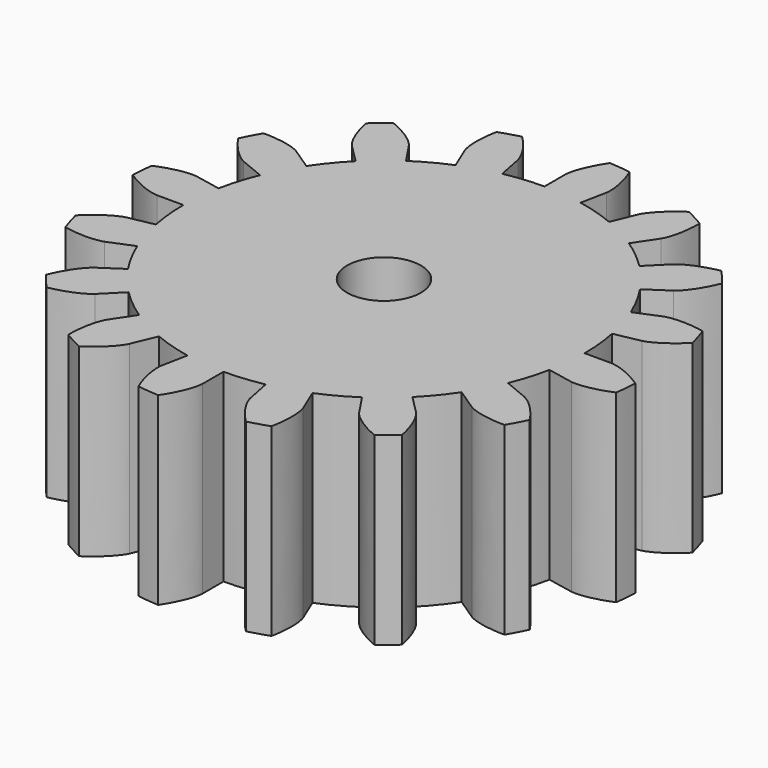
from build123d import *

# Parameters (mm, degrees)
F3_DEPTH        = 8
F3_COPIES_COUNT = 16
F5_R            = 1.6
F6_DEPTH        = 25


# Not quite as in the source:
# - a feature of the source that left no trace in its solid (it failed there, or was rolled back) is left out
# - a pattern or mirror of a feature is missing from the dataset's text; its kind, count and spacing are read off the source's solid
# - a feature names something its author has since deleted; it is built from what else it names


with BuildPart() as f3:
    # F2 (on Top) → F3 (new body)
    with BuildSketch(Plane.XY):
        with BuildLine():
            ThreePointArc((-8.69061, 0), (0, -8.69061), (8.69061, 0))
            ThreePointArc((8.69061, 0), (0.8518287399, 8.6487623375), (-8.5236223657, 1.6954539034))
            ThreePointArc((-8.5236223657, 1.6954539034), (-8.6487623375, 0.8518287399), (-8.69061, 0))
        make_face()
        with BuildLine():
            ThreePointArc((-8.69061, 0), (-8.6487623375, 0.8518287399), (-8.5236223657, 1.6954539034))
            Line((-8.5236223657, 1.6954539034), (-9.6473767422, 1.9189825468))
            add(Edge.make_bspline(
                [(-9.6473767422, 1.9189825468), (-9.6530150918, 1.9201040843), (-9.6588355491, 1.9209090828), (-9.6997192411, 1.9262346758), (-9.7590494013, 1.9302321469), (-9.8457579233, 1.9321979419), (-9.9561731199, 1.928983786), (-10.0911078559, 1.9183660608), (-10.2496444634, 1.8978526592), (-10.4312304204, 1.8650534214), (-10.6347503632, 1.8177279697), (-10.8599182557, 1.7531773691), (-11.0878990517, 1.6758254952), (-11.2481946283, 1.6121629894), (-11.3199310277, 1.5824226766)],
                knots=[0, 0, 0, 0, 0.0202164122, 0.055231725, 0.1004362437, 0.1539229332, 0.2145711301, 0.2816202297, 0.3545102827, 0.4328067574, 0.5161597183, 0.6042794907, 0.6969211254, 0.7772832798, 0.7772832798, 0.7772832798, 0.7772832798], degree=3))
            ThreePointArc((-11.3199310277, 1.5824226766), (-11.3749614259, 1.120335914), (-11.4111370767, 0.6563921208))
            add(Edge.make_bspline(
                [(-9.8363800262, 0), (-9.8421288376, 0), (-9.8479945039, 0.0003459841), (-9.8891315989, 0.0030987336), (-9.9481016147, 0.0107528128), (-10.0335275643, 0.0257407835), (-10.1411941132, 0.0504341165), (-10.2714647006, 0.0871722862), (-10.4229531055, 0.1382204864), (-10.5946511254, 0.2058151589), (-10.7850277519, 0.2919360364), (-10.993275909, 0.399174392), (-11.201785516, 0.5195168183), (-11.3465811193, 0.6132281825), (-11.4111370767, 0.6563921208)],
                knots=[0, 0, 0, 0, 0.0202164122, 0.055231725, 0.1004362437, 0.1539229332, 0.2145711301, 0.2816202297, 0.3545102827, 0.4328067574, 0.5161597183, 0.6042794907, 0.6969211254, 0.7772832798, 0.7772832798, 0.7772832798, 0.7772832798], degree=3))
            Line((-9.8363800262, 0), (-8.69061, 0))
        make_face()
    extrude(amount=F3_DEPTH)

    # F3_copies: F3 ×16 about axis
    f3_copies_axis = Axis((0, 0, 0), (0, 0, 1))


with BuildPart() as f3_1:
    add(f3.part)
    for i in range(1, F3_COPIES_COUNT):
        add(f3.part.rotate(f3_copies_axis, i * 360 / F3_COPIES_COUNT))

    # F5 (on face) → F6 (cut)
    with BuildSketch(Plane.XY.offset(8)):
        Circle(F5_R)
    extrude(amount=-F6_DEPTH, mode=Mode.SUBTRACT)


solid = f3_1.part
